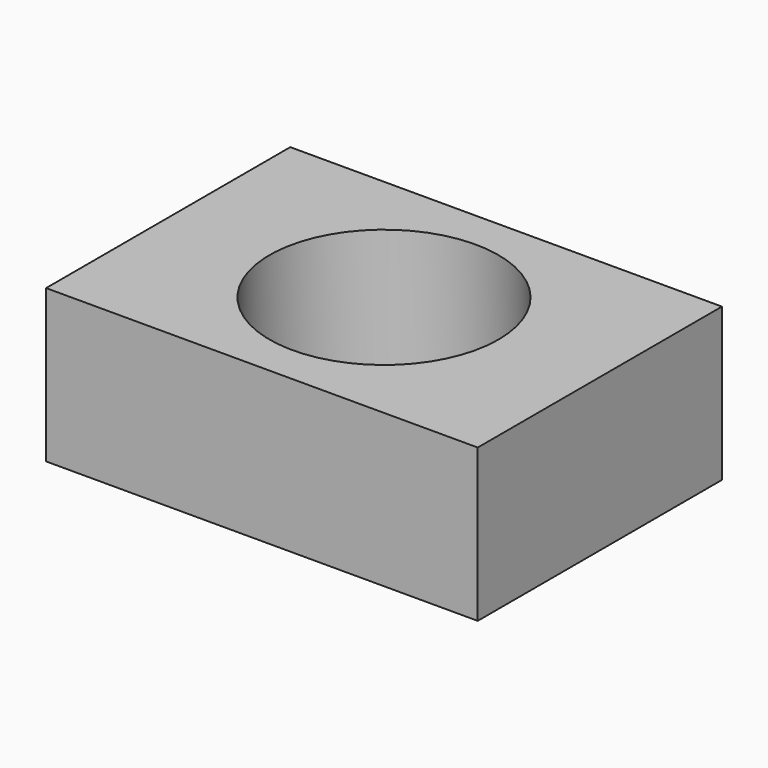
from build123d import *

# Parameters (mm, degrees)
F0_W     = 35.9210356
F0_H     = 12.7
F1_DEPTH = 12.7
F2_R     = 9.525
F3_DEPTH = 12.701


# Not quite as in the source:
# - the program builds the solid bodies; features that only make, move or delete a surface that nothing else refers to are left out


with BuildPart() as f1:
    # F0 (on Front) → F1 (new body, symmetric)
    with BuildSketch(Plane.XZ):
        Rectangle(F0_W, F0_H)
    extrude(amount=F1_DEPTH, both=True)

    # F2 (on face) → F3 (cut, through all)
    with BuildSketch(Plane.XY.offset(6.35)):
        Circle(F2_R)
    extrude(amount=-F3_DEPTH, mode=Mode.SUBTRACT)


solid = f1.part
